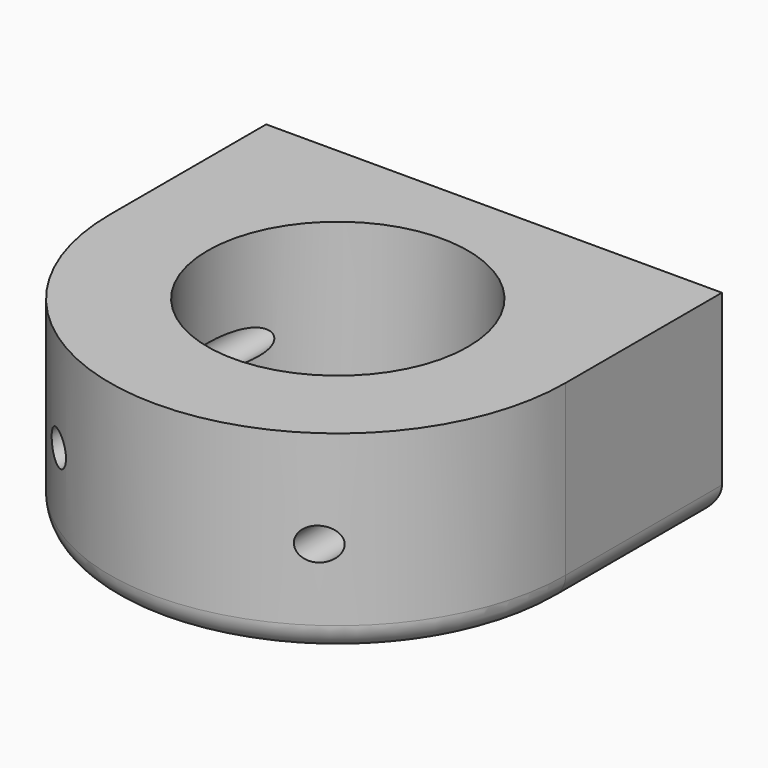
from build123d import *

# Parameters (mm, degrees)
F0_R         = 25.4
F1_DEPTH     = 38.1
F2_R         = 3.175
F3_DEPTH     = 96.774
F4_R         = 6.35
F4_R_2       = 3.175
F5_DEPTH     = 7.366
F6_R         = 5.08
F7_TEXT_SIZE = 15.2524521885
F8_DEPTH     = 5.588


# Not quite as in the source:
# - Text() gives the source's letters only with a copy of the font that has no kerning and outlines rounded to 1/6400 em; it was checked with that copy


with BuildPart() as f1:
    # F0 (on Top) → F1 (new body)
    with BuildSketch(Plane.XY):
        with BuildLine():
            Line((-44.45, 38.1), (-44.45, 0))
            ThreePointArc((-44.45, 0), (0, -44.45), (44.45, 0))
            Line((44.45, 0), (44.45, 38.1))
            Line((44.45, 38.1), (-44.45, 38.1))
        make_face()
        Circle(F0_R, mode=Mode.SUBTRACT)
    extrude(amount=F1_DEPTH)

    # F2 (on face) → F3 (cut)
    with BuildSketch(Plane(origin=(0, 38.1, 0), x_dir=(-1, 0, 0), z_dir=(0, 1, 0))):
        with Locations((-25.4, 19.05)):
            Circle(F2_R)
        with Locations((25.4, 19.05)):
            Circle(F2_R)
    extrude(amount=-F3_DEPTH, mode=Mode.SUBTRACT)

    # F4 (on face) → F5 (cut)
    with BuildSketch(Plane(origin=(0, 38.1, 0), x_dir=(-1, 0, 0), z_dir=(0, 1, 0))):
        with Locations((-25.4, 19.05)):
            Circle(F4_R)
        with Locations((-25.4, 19.05)):
            Circle(F4_R_2, mode=Mode.SUBTRACT)
        with Locations((25.4, 19.05)):
            Circle(F4_R)
        with Locations((25.4, 19.05)):
            Circle(F4_R_2, mode=Mode.SUBTRACT)
    extrude(amount=-F5_DEPTH, mode=Mode.SUBTRACT)

    # F6
    f6_edges = [f1.edges().sort_by_distance(p)[0] for p in [
        (44.45, 19.05, 0),
        (0, 38.1, 0),
        (-44.45, 19.05, 0),
        (0, -44.45, 0),
        (-25.4, 0, 0),
    ]]
    fillet(f6_edges, radius=F6_R)

    # F7 (on face) → F8 (cut)
    with BuildSketch(Plane(origin=(0, 38.1, 0), x_dir=(-1, 0, 0), z_dir=(0, 1, 0))):
        with Locations((-8.5164699703, 9.6370587125)):
            Text('haha', F7_TEXT_SIZE, font='Tinos', font_style=FontStyle.BOLD, text_align=(TextAlign.LEFT, TextAlign.BOTTOM))
    extrude(amount=-F8_DEPTH, mode=Mode.SUBTRACT)


solid = f1.part
